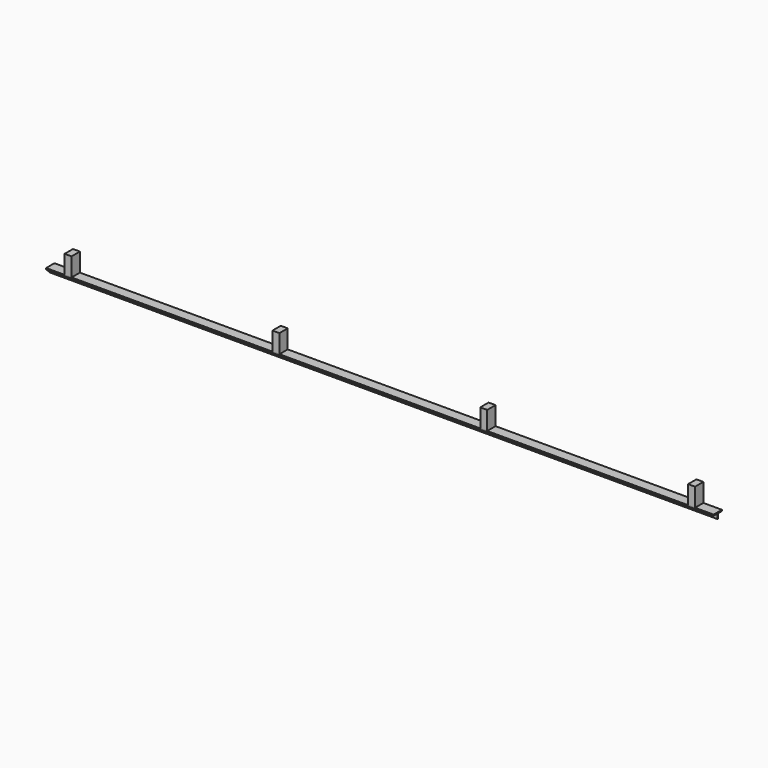
from build123d import *

# Parameters (mm, degrees)
F0_W     = 1828.8
F0_H     = 28.575
F1_DEPTH = 3.175
F4_W     = 19.05
F4_H     = 28.575
F5_DEPTH = 50.8
F6_W     = 1828.8
F6_H     = 3.175
F7_DEPTH = 12.7
F9_DEPTH = 3.175


# Not quite as in the source:
# - a feature of the source that left no trace in its solid (it failed there, or was rolled back) is left out


with BuildPart() as f1:
    # F0 (on Top) → F1 (new body)
    with BuildSketch(Plane.XY):
        with Locations((-914.4, 14.2875)):
            Rectangle(F0_W, F0_H)
    extrude(amount=F1_DEPTH)

    # F6 (on face) → F7 (join)
    with BuildSketch(Plane(origin=(0, 0, 0), x_dir=(1, 0, 0), z_dir=(0, 0, -1))):
        with Locations((-914.4, -14.2875)):
            Rectangle(F6_W, F6_H)
    extrude(amount=F7_DEPTH)


with BuildPart() as f5:
    # F4 (on face) → F5 (new body)
    with BuildSketch(Plane.XY.offset(3.175)):
        with Locations((-1768.475, 14.2875)):
            Rectangle(F4_W, F4_H)
    extrude(amount=F5_DEPTH)


with BuildPart() as f5b:
    # F4 (on face) → F5, piece 2 (new body)
    with BuildSketch(Plane.XY.offset(3.175)):
        with Locations((-1199.0916666667, 14.2875)):
            Rectangle(F4_W, F4_H)
    extrude(amount=F5_DEPTH)


with BuildPart() as f5c:
    # F4 (on face) → F5, piece 3 (new body)
    with BuildSketch(Plane.XY.offset(3.175)):
        with Locations((-629.7083333333, 14.2875)):
            Rectangle(F4_W, F4_H)
    extrude(amount=F5_DEPTH)


with BuildPart() as f5d:
    # F4 (on face) → F5, piece 4 (new body)
    with BuildSketch(Plane.XY.offset(3.175)):
        with Locations((-60.325, 14.2875)):
            Rectangle(F4_W, F4_H)
    extrude(amount=F5_DEPTH)


with BuildPart() as f9:
    # F8 (on face) → F9 (new body)
    with BuildSketch(Plane(origin=(-1828.8, 0, 0), x_dir=(0, -1, 0), z_dir=(-1, 0, 0))):
        Polygon((-12.7, -12.7), (0, 0), (-12.7, 0), align=None)
    extrude(amount=-F9_DEPTH)


with BuildPart() as f9b:
    # F8 (on face) → F9, piece 2 (new body)
    with BuildSketch(Plane(origin=(-1828.8, 0, 0), x_dir=(0, -1, 0), z_dir=(-1, 0, 0))):
        Polygon((-28.575, 0), (-15.875, -12.7), (-15.875, 0), align=None)
    extrude(amount=-F9_DEPTH)


solid = Compound([f1.part, f5.part, f5b.part, f5c.part, f5d.part, f9.part, f9b.part])
